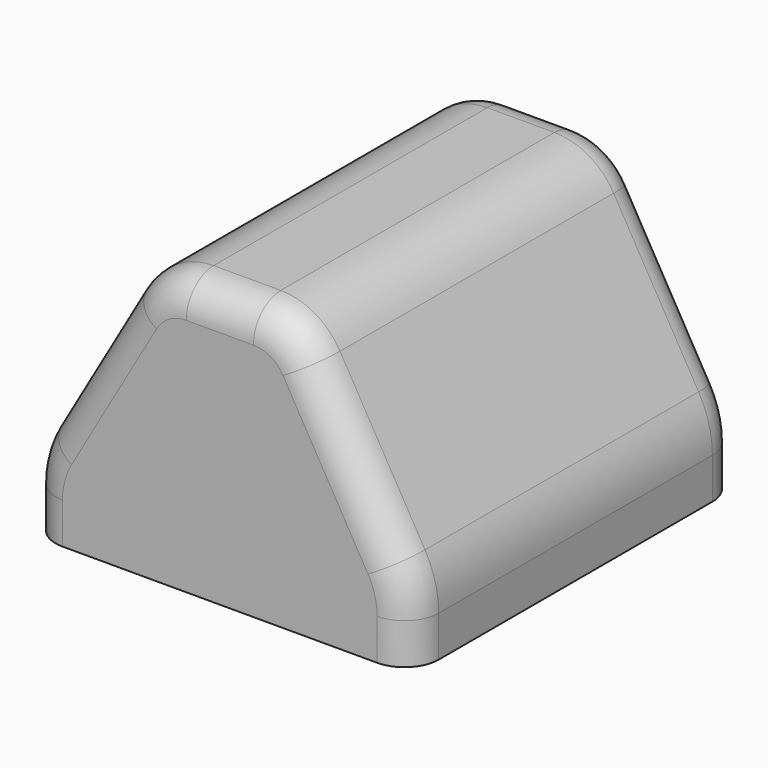
from build123d import *

# Parameters (mm, degrees)
F0_W     = 112
F0_H     = 120
F1_DEPTH = 20
F2_DEPTH = 60
F3_SIZE2 = 34.641006
F3_SIZE  = 59.99999
F4_SIZE2 = 34.641006
F4_SIZE  = 59.99999
F5_R     = 20
F7_R     = 30
F8_R     = 10


# Not quite as in the source:
# - a fillet or chamfer is up to 0.001 mm smaller than in the source, because OpenCascade refuses the exact size


with BuildPart() as f1:
    # F0 (on Top) → F1 (new body)
    with BuildSketch(Plane.XY):
        with Locations((0.0172033906, -34.0157587473)):
            Rectangle(F0_W, F0_H)
    extrude(amount=F1_DEPTH)


with BuildPart() as f2:
    # F2 (new): a face of the model
    f2_faces = [f1.part.faces().sort_by_distance(p)[0] for p in [
        (0.0172033906, -34.0157587473, 20),
    ]]
    extrude(f2_faces, amount=F2_DEPTH)

    # F3 (size 60 and 34.6410161514 in the source; OpenCascade refuses exactly that, so slightly less here)
    f3_edges = [f2.edges().sort_by_distance(p)[0] for p in [
        (56.017203, -34.015759, 80),
    ]]
    f3_side = f2.faces().sort_by_distance((56.017203, -34.015759, 50))[0]
    chamfer(f3_edges, length=F3_SIZE, length2=F3_SIZE2, reference=f3_side)

    # F4 (size 60 and 34.6410161514 in the source; OpenCascade refuses exactly that, so slightly less here)
    f4_edges = [f2.edges().sort_by_distance(p)[0] for p in [
        (-55.982797, -34.015759, 80),
    ]]
    f4_side = f2.faces().sort_by_distance((-55.982797, -34.015759, 50))[0]
    chamfer(f4_edges, length=F4_SIZE, length2=F4_SIZE2, reference=f4_side)

    # F5
    f5_edges = [f2.edges().sort_by_distance(p)[0] for p in [
        (21.376197, -34.015759, 80),
        (-21.341791, -34.015759, 80),
    ]]
    fillet(f5_edges, radius=F5_R)


with BuildPart() as f1_1:
    add(f1.part)

    # F6: union F2
    add(f2.part)

    # F7
    f7_edges = [f1_1.edges().sort_by_distance(p)[0] for p in [
        (-55.982797, -34.015759, 20),
        (56.017203, -34.015759, 20),
    ]]
    fillet(f7_edges, radius=F7_R)

    # F8
    f8_edges = [f1_1.edges().sort_by_distance(p)[0] for p in [
        (-39.539426, -94.015759, 48.480766),
        (-55.982797, -94.015759, 5.980768),
        (-39.539426, 25.984241, 48.480766),
        (-55.982797, 25.984241, 5.980768),
    ]]
    fillet(f8_edges, radius=F8_R)


solid = f1_1.part
